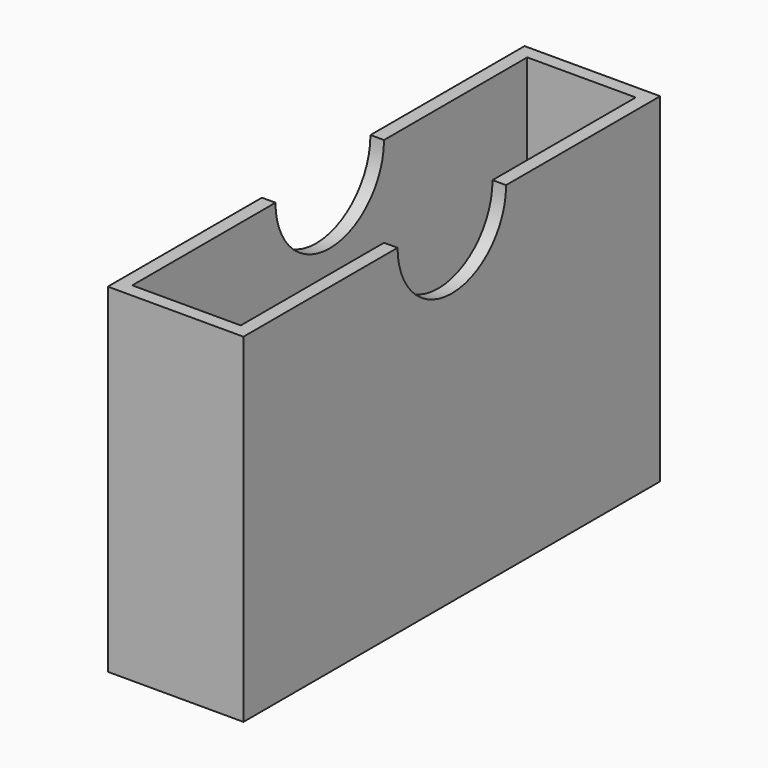
from build123d import *

# Parameters (mm, degrees)
F0_W     = 20
F0_H     = 91
F1_DEPTH = 60
F2_T     = 2.5
F4_DEPTH = 25.001


with BuildPart() as f1:
    # F0 (on Top) → F1 (new body)
    with BuildSketch(Plane.XY):
        Rectangle(F0_W, F0_H)
    extrude(amount=F1_DEPTH)

    # F2
    f2_openings = [f1.faces().sort_by_distance(p)[0] for p in [
        (0, 0, 60),
    ]]
    offset(amount=F2_T, openings=f2_openings, kind=Kind.INTERSECTION)

    # F3 (on face) → F4 (cut, through all)
    with BuildSketch(Plane.YZ.offset(12.5)):
        with BuildLine():
            ThreePointArc((-12.5, 60), (0, 47.5), (12.5, 60))
            Line((12.5, 60), (-12.5, 60))
        make_face()
    extrude(amount=-F4_DEPTH, mode=Mode.SUBTRACT)


solid = f1.part
